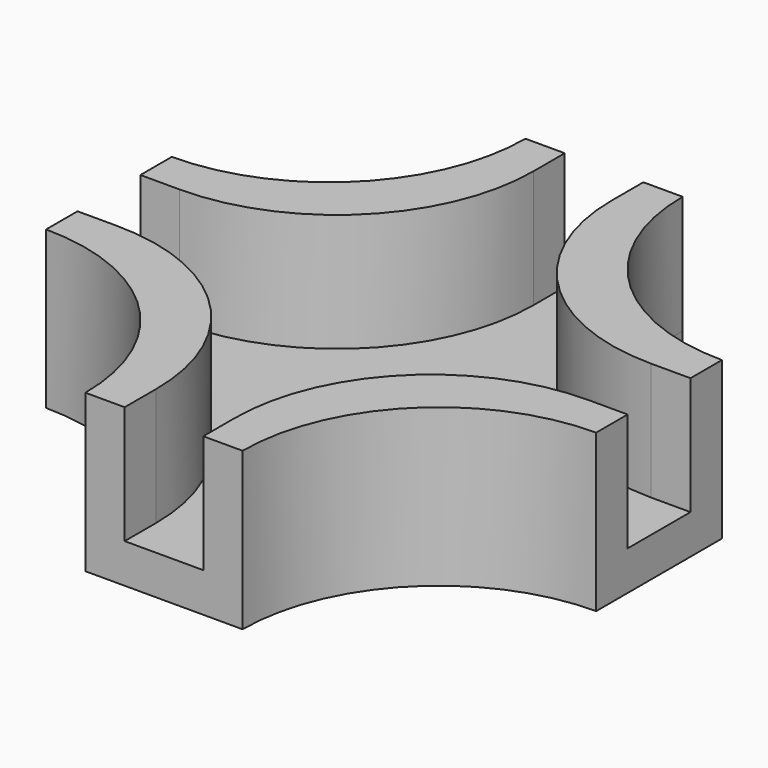
from build123d import *

# Parameters (mm, degrees)
F0_W     = 14
F0_H     = 14
F1_DEPTH = 1
F2_W     = 5
F2_H     = 1
F3_DEPTH = 3
F4_R     = 4.99999
F5_DEPTH = 25


# Not quite as in the source:
# - a fillet or chamfer is up to 0.001 mm smaller than in the source, because OpenCascade refuses the exact size


with BuildPart() as f1:
    # F0 (on Top) → F1 (new body)
    with BuildSketch(Plane.XY):
        Rectangle(F0_W, F0_H)
    extrude(amount=F1_DEPTH)

    # F2 (on face) → F3 (join)
    with BuildSketch(Plane.XY.offset(1)):
        Polygon((-1, 1), (-1, 7), (-2, 7), (-2, 2), (-2, 1), align=None)
        with Locations((-4.5, 1.5)):
            Rectangle(F2_W, F2_H)
        Polygon((1, 1), (2, 1), (2, 2), (2, 7), (1, 7), align=None)
        with Locations((4.5, 1.5)):
            Rectangle(F2_W, F2_H)
        with Locations((4.5, -1.5)):
            Rectangle(F2_W, F2_H)
        Polygon((2, -1), (1, -1), (1, -7), (2, -7), (2, -2), align=None)
        with Locations((-4.5, -1.5)):
            Rectangle(F2_W, F2_H)
        Polygon((-2, -7), (-1, -7), (-1, -1), (-2, -1), (-2, -2), align=None)
    extrude(amount=F3_DEPTH)

    # F4 (radius 5 in the source; OpenCascade refuses exactly that, so slightly less here)
    f4_edges = [f1.edges().sort_by_distance(p)[0] for p in [
        (2, -2, 2.5),
        (-1, -1, 2.5),
        (-1, 1, 2.5),
        (1, 1, 2.5),
        (2, 2, 2.5),
        (-2, 2, 2.5),
        (-2, -2, 2.5),
        (1, -1, 2.5),
    ]]
    fillet(f4_edges, radius=F4_R)

    # F5 (cut): faces of the model
    f5_faces = [f1.faces().sort_by_distance(p)[0] for p in [
        (4.8779327776, -4.8779327776, 1),
        (4.8779327776, 4.8779327776, 1),
        (-4.8779327776, 4.8779327776, 1),
        (-4.8779327776, -4.8779327776, 1),
    ]]
    extrude(f5_faces, amount=-F5_DEPTH, mode=Mode.SUBTRACT)


solid = f1.part
